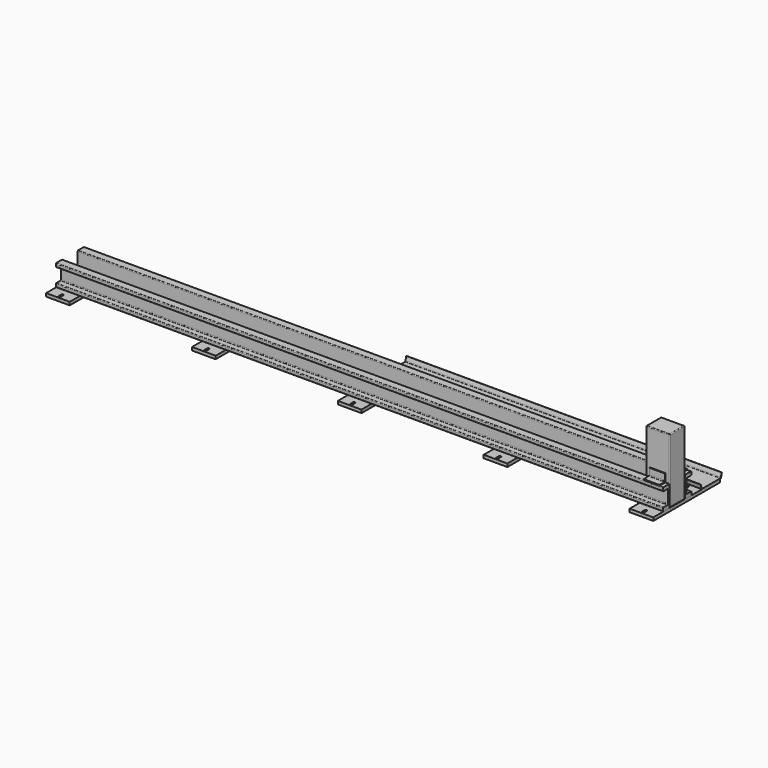
from build123d import *

# Parameters (mm, degrees)
F0_W      = 150
F0_H      = 380
F1_DEPTH  = 20
F3_DEPTH  = 1925
F5_DEPTH  = 2000
F6_W      = 150
F6_H      = 120
F7_DEPTH  = 410
F8_R      = 5
F9_R      = 5
F12_DEPTH = 50


with BuildPart() as f1:
    # F0 (on Top) → F1 (new body)
    with BuildSketch(Plane.XY):
        with Locations((-1850, 0)):
            Rectangle(F0_W, F0_H)
        with BuildLine():
            ThreePointArc((-1843, -175), (-1850, -182), (-1857, -175))
            Line((-1857, -175), (-1857, -155))
            ThreePointArc((-1857, -155), (-1850, -148), (-1843, -155))
            Line((-1843, -155), (-1843, -175))
        make_face(mode=Mode.SUBTRACT)
        with BuildLine():
            Line((-1857, 155), (-1857, 175))
            ThreePointArc((-1857, 175), (-1850, 182), (-1843, 175))
            Line((-1843, 175), (-1843, 155))
            ThreePointArc((-1843, 155), (-1850, 148), (-1857, 155))
        make_face(mode=Mode.SUBTRACT)
    extrude(amount=-F1_DEPTH)


with BuildPart() as f1b:
    # F0 (on Top) → F1, piece 2 (new body)
    with BuildSketch(Plane.XY):
        with Locations((-925, 0)):
            Rectangle(F0_W, F0_H)
        with BuildLine():
            ThreePointArc((-918, -175), (-925, -182), (-932, -175))
            Line((-932, -175), (-932, -155))
            ThreePointArc((-932, -155), (-925, -148), (-918, -155))
            Line((-918, -155), (-918, -175))
        make_face(mode=Mode.SUBTRACT)
        with BuildLine():
            Line((-932, 155), (-932, 175))
            ThreePointArc((-932, 175), (-925, 182), (-918, 175))
            Line((-918, 175), (-918, 155))
            ThreePointArc((-918, 155), (-925, 148), (-932, 155))
        make_face(mode=Mode.SUBTRACT)
    extrude(amount=-F1_DEPTH)


with BuildPart() as f1c:
    # F0 (on Top) → F1, piece 3 (new body)
    with BuildSketch(Plane.XY):
        Polygon((-75, 190), (-75, -190), (75, -190), (75, 190), (75, 340), (-75, 340), align=None)
        with BuildLine():
            ThreePointArc((7, -175), (0, -182), (-7, -175))
            Line((-7, -175), (-7, -155))
            ThreePointArc((-7, -155), (0, -148), (7, -155))
            Line((7, -155), (7, -175))
        make_face(mode=Mode.SUBTRACT)
        with BuildLine():
            Line((-7, 155), (-7, 175))
            ThreePointArc((-7, 175), (0, 182), (7, 175))
            Line((7, 175), (7, 155))
            ThreePointArc((7, 155), (0, 148), (-7, 155))
        make_face(mode=Mode.SUBTRACT)
    extrude(amount=-F1_DEPTH)

    # F2 (on Right) → F3 (join, symmetric)
    with BuildSketch(Plane.YZ):
        with BuildLine():
            ThreePointArc((-113, 5), (-111.5355339059, 1.4644660941), (-108, 0))
            Line((-108, 0), (-65, 0))
            ThreePointArc((-65, 0), (-61.4644660941, 1.4644660941), (-60, 5))
            Line((-60, 5), (-60, 130.5))
            ThreePointArc((-60, 130.5), (-61.4644660941, 134.0355339059), (-65, 135.5))
            Line((-65, 135.5), (-108, 135.5))
            ThreePointArc((-108, 135.5), (-111.5355339059, 134.0355339059), (-113, 130.5))
            Line((-113, 130.5), (-113, 117.5))
            ThreePointArc((-113, 117.5), (-111.5355339059, 113.9644660941), (-108, 112.5))
            Line((-108, 112.5), (-77.5, 112.5))
            ThreePointArc((-77.5, 112.5), (-73.9644660941, 111.0355339059), (-72.5, 107.5))
            Line((-72.5, 107.5), (-72.5, 28))
            ThreePointArc((-72.5, 28), (-73.9644660941, 24.4644660941), (-77.5, 23))
            Line((-77.5, 23), (-108, 23))
            ThreePointArc((-108, 23), (-111.5355339059, 21.5355339059), (-113, 18))
            Line((-113, 18), (-113, 5))
        make_face()
        with BuildLine():
            ThreePointArc((65, 135.5), (61.4644660941, 134.0355339059), (60, 130.5))
            Line((60, 130.5), (60, 5))
            ThreePointArc((60, 5), (61.4644660941, 1.4644660941), (65, 0))
            Line((65, 0), (108, 0))
            ThreePointArc((108, 0), (111.5355339059, 1.4644660941), (113, 5))
            Line((113, 5), (113, 18))
            ThreePointArc((113, 18), (111.5355339059, 21.5355339059), (108, 23))
            Line((108, 23), (77.5, 23))
            ThreePointArc((77.5, 23), (73.9644660941, 24.4644660941), (72.5, 28))
            Line((72.5, 28), (72.5, 107.5))
            ThreePointArc((72.5, 107.5), (73.9644660941, 111.0355339059), (77.5, 112.5))
            Line((77.5, 112.5), (108, 112.5))
            ThreePointArc((108, 112.5), (111.5355339059, 113.9644660941), (113, 117.5))
            Line((113, 117.5), (113, 130.5))
            ThreePointArc((113, 130.5), (111.5355339059, 134.0355339059), (108, 135.5))
            Line((108, 135.5), (65, 135.5))
        make_face()
    extrude(amount=F3_DEPTH, both=True)


with BuildPart() as f1d:
    # F0 (on Top) → F1, piece 4 (new body)
    with BuildSketch(Plane.XY):
        Polygon((850, 190), (850, -190), (1000, -190), (1000, 190), (1000, 340), (850, 340), align=None)
        with BuildLine():
            ThreePointArc((932, -175), (925, -182), (918, -175))
            Line((918, -175), (918, -155))
            ThreePointArc((918, -155), (925, -148), (932, -155))
            Line((932, -155), (932, -175))
        make_face(mode=Mode.SUBTRACT)
        with BuildLine():
            Line((918, 155), (918, 175))
            ThreePointArc((918, 175), (925, 182), (932, 175))
            Line((932, 175), (932, 155))
            ThreePointArc((932, 155), (925, 148), (918, 155))
        make_face(mode=Mode.SUBTRACT)
    extrude(amount=-F1_DEPTH)


with BuildPart() as f1e:
    # F0 (on Top) → F1, piece 5 (new body)
    with BuildSketch(Plane.XY):
        Polygon((1775, 190), (1775, -190), (1925, -190), (1925, 190), (1925, 340), (1775, 340), align=None)
        with BuildLine():
            ThreePointArc((1857, -175), (1850, -182), (1843, -175))
            Line((1843, -175), (1843, -155))
            ThreePointArc((1843, -155), (1850, -148), (1857, -155))
            Line((1857, -155), (1857, -175))
        make_face(mode=Mode.SUBTRACT)
        with BuildLine():
            Line((1843, 155), (1843, 175))
            ThreePointArc((1843, 175), (1850, 182), (1857, 175))
            Line((1857, 175), (1857, 155))
            ThreePointArc((1857, 155), (1850, 148), (1843, 155))
        make_face(mode=Mode.SUBTRACT)
    extrude(amount=-F1_DEPTH)


with BuildPart() as f5:
    # F4 (on face) → F5 (new body, through all)
    with BuildSketch(Plane.YZ.offset(1925)):
        with BuildLine():
            Line((347.8255626562, 5.3022506247), (354, 30))
            Line((354, 30), (352.0597149997, 30.4850712501))
            Line((352.0597149997, 30.4850712501), (345.8852776559, 5.7873218748))
            ThreePointArc((345.8852776559, 5.7873218748), (344.1116262022, 3.0589728099), (341.0345651552, 2))
            Line((341.0345651552, 2), (269.5, 2))
            Line((269.5, 2), (197.9654348448, 2))
            ThreePointArc((197.9654348448, 2), (194.8883737978, 3.0589728099), (193.1147223441, 5.7873218748))
            Line((193.1147223441, 5.7873218748), (186.9402850003, 30.4850712501))
            Line((186.9402850003, 30.4850712501), (185, 30))
            Line((185, 30), (191.1744373438, 5.3022506247))
            ThreePointArc((191.1744373438, 5.3022506247), (193.657549379, 1.4825619339), (197.9654348448, 0))
            Line((197.9654348448, 0), (269.5, 0))
            Line((269.5, 0), (341.0345651552, 0))
            ThreePointArc((341.0345651552, 0), (345.342450621, 1.4825619339), (347.8255626562, 5.3022506247))
        make_face()
    extrude(amount=-F5_DEPTH)


with BuildPart() as f7:
    # F6 (on face) → F7 (new body)
    with BuildSketch(Plane.XY):
        with Locations((1850, 0)):
            Rectangle(F6_W, F6_H)
    extrude(amount=F7_DEPTH)

    # F8
    f8_edges = [f7.edges().sort_by_distance(p)[0] for p in [
        (1925, -60, 205),
        (1775, -60, 205),
        (1925, 60, 205),
        (1775, 60, 205),
        (1925, 0, 410),
        (1850, 60, 410),
        (1775, 0, 410),
        (1850, -60, 410),
    ]]
    fillet(f8_edges, radius=F8_R)

    # F9
    f9_edges = [f7.edges().sort_by_distance(p)[0] for p in [
        (1925, 0, 0),
        (1925, -55, 202.5),
        (1925, 55, 202.5),
        (1925, 0, 405),
    ]]
    fillet(f9_edges, radius=F9_R)


with BuildPart() as f12:
    # F11 (on offset) → F12 (new body, symmetric)
    with BuildSketch(Plane.YZ.offset(1850)):
        with BuildLine():
            Line((-63.6203959584, 135.5), (-60, 135.5))
            Line((-60, 135.5), (-60, 185.5))
            Line((-60, 185.5), (-65, 185.5))
            Line((-65, 185.5), (-65, 145.5))
            ThreePointArc((-65, 145.5), (-66.4644660941, 141.9644660941), (-70, 140.5))
            Line((-70, 140.5), (-110, 140.5))
            Line((-110, 140.5), (-110, 135.5))
            Line((-110, 135.5), (-108, 135.5))
            Line((-108, 135.5), (-63.6203959584, 135.5))
        make_face()
    extrude(amount=F12_DEPTH, both=True)


with BuildPart() as f13_1:
    # F13: instance of F12
    add(f12.part.mirror(Plane.XZ))


solid = Compound([f1.part, f1b.part, f1c.part, f1d.part, f1e.part, f5.part, f7.part, f12.part, f13_1.part])
